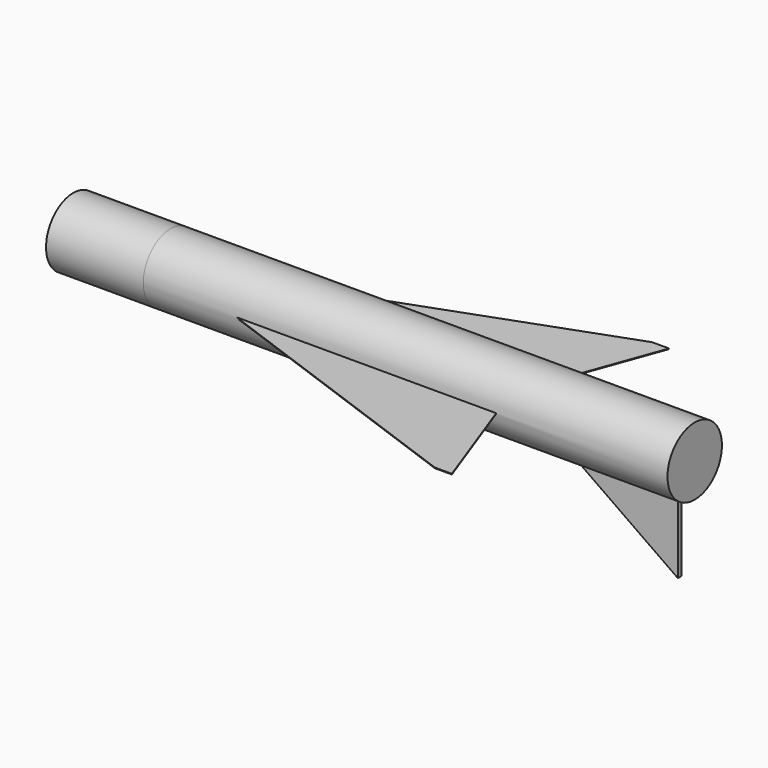
from build123d import *

# Parameters (mm, degrees)
F1_DEPTH = 12.7
F3_R     = 1400
F4_DEPTH = 21569
F5_DEPTH = 4000
F9_DEPTH = 100


# Not quite as in the source:
# - the program builds the solid bodies; features that only make, move or delete a surface that nothing else refers to are left out


with BuildPart() as f1:
    # F0 (on Top) → F1 (new body, symmetric)
    with BuildSketch(Plane.XY):
        Polygon((15344.7909177956, 5585.047145116), (0, 0), (14012, 0), (16044.7909177956, 5585.047145116), align=None)
    extrude(amount=F1_DEPTH, both=True)

    # F2: F1 across plane


with BuildPart() as f1_1:
    add(f1.part)
    add(f1.part.mirror(Plane.XZ))

    # F3 (on Right) → F4 (join)
    with BuildSketch(Plane.YZ):
        Circle(F3_R)
    extrude(amount=F4_DEPTH)

    # F3 (on Right) → F5 (join)
    with BuildSketch(Plane.YZ):
        Circle(F3_R)
    extrude(amount=-F5_DEPTH)

    # F8 (on Front) → F9 (join, symmetric)
    with BuildSketch(Plane.XZ):
        Polygon((16683.6071014404, -1400), (20955.2135467529, -4400), (20955.2135467529, -1400), align=None)
    extrude(amount=F9_DEPTH, both=True)


solid = f1_1.part
